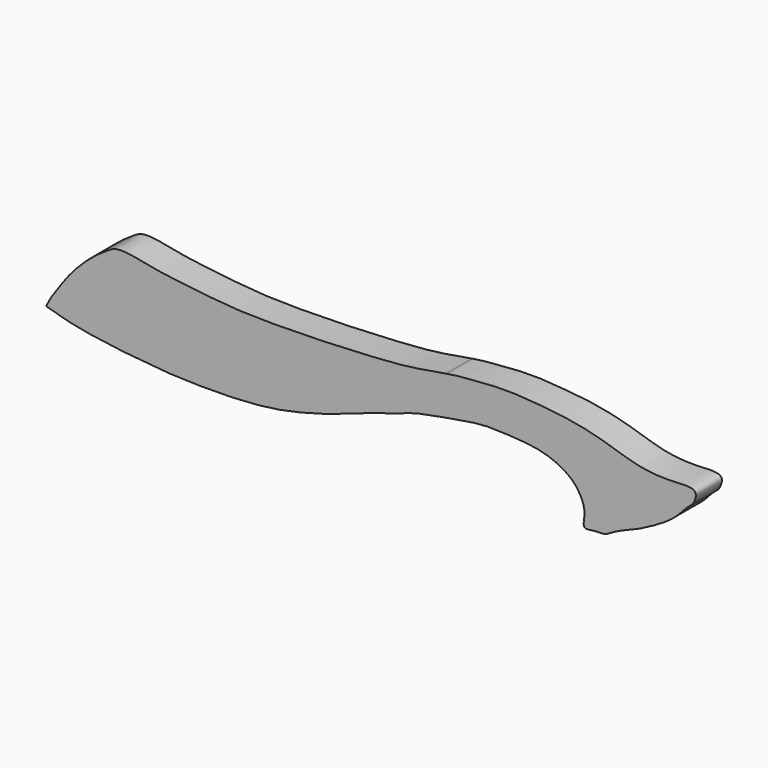
from build123d import *

# Parameters (mm, degrees)
F1_DEPTH = 25.4


with BuildPart() as f1:
    # F0 (on Front) → F1 (new body)
    with BuildSketch(Plane.XZ):
        with BuildLine():
            add(Edge.make_bspline(
                [(-41.3323794244, 51.0675903058), (-41.707539983, 51.0071643032), (-42.0874786851, 50.9453207608), (-42.4716510296, 50.8822327158)],
                knots=[0.7233820323, 0.7233820323, 0.7233820323, 0.7233820323, 0.7244841774, 0.7244841774, 0.7244841774, 0.7244841774], degree=3))
            Line((-42.4716510296, 50.8822327158), (-42.4716510296, 20.6025924894))
            add(Edge.make_bspline(
                [(-42.4716510296, 20.6025924894), (-38.0350865118, 21.387674424), (-27.1703671298, 23.2609805149), (-11.8336777596, 25.6290338302), (6.2117415006, 24.6446677805), (22.8981387265, 23.7685028967), (40.3803315985, 20.265824034), (56.0268632555, 11.4827913687), (63.3288722201, 1.5132508922), (67.2395318395, -9.5186102569), (63.4930685042, -21.7540557946), (73.9984795886, -18.6916156231), (82.1685298982, -19.9874563616), (89.9568581577, -13.8368079067), (103.8859155375, -9.029814598), (115.48254286, -3.1488551069), (127.3676268383, 3.4775298147), (138.3862701068, 11.274252363), (146.0514505158, 21.0054750541), (150.7100984849, 23.1711418755), (154.3469370428, 32.4931326622), (147.7952194183, 35.6662775706), (131.9063905367, 33.9551189768), (113.1540349234, 35.1939826272), (98.5720074401, 38.9368599863), (80.3169366587, 45.0640141502), (58.980025117, 50.1412876611), (38.6431779668, 52.6423918075), (18.2586858505, 54.3804757709), (-2.1281200842, 55.0935858146), (-25.7150036655, 52.83496744), (-33.7024906401, 52.247249559), (-39.6317656905, 51.3415031345), (-41.3323794244, 51.0675903058)],
                knots=[0.2661930696, 0.2661930696, 0.2661930696, 0.2661930696, 0.2780888488, 0.2952566157, 0.3124048676, 0.3290318413, 0.3462265461, 0.3632256959, 0.3773149803, 0.3913700519, 0.4035868461, 0.4147193685, 0.4265046687, 0.4388744688, 0.4544742419, 0.4692690904, 0.4841731354, 0.4993562758, 0.5132863243, 0.5226012229, 0.5341358793, 0.5434033522, 0.5596575999, 0.5774651553, 0.5931774764, 0.6109205173, 0.6300378187, 0.6484766733, 0.6666946566, 0.6854295214, 0.7048957488, 0.7183859765, 0.7233820323, 0.7233820323, 0.7233820323, 0.7233820323], degree=3))
        make_face()
        with BuildLine():
            Line((-42.4716510296, 20.6025924894), (-42.4716510296, 50.8822327158))
            add(Edge.make_bspline(
                [(-42.4716510296, 50.8822327158), (-46.5466181639, 50.2130494346), (-58.4983628647, 48.0880744628), (-77.3183947596, 45.1720060107), (-109.6591600511, 43.2576521666), (-142.7930612804, 41.7374006357), (-176.1120717601, 41.1768442804), (-208.717867936, 41.5632407424), (-242.6772032351, 45.6151659887), (-270.6437105384, 48.6410725006), (-297.2774912922, 55.186574868), (-306.7493706772, 49.342600006), (-316.6435316034, 42.6087777486), (-327.9751917318, 32.5628982927), (-337.3736197705, 21.5291356577), (-343.7111475225, 12.5988365582), (-348.0439396481, 6.508227293), (-349.970638752, 3.5016264301)],
                knots=[0.7244841774, 0.7244841774, 0.7244841774, 0.7244841774, 0.7361747771, 0.7551837741, 0.7782030276, 0.8018366623, 0.8252292117, 0.8485245896, 0.8721716095, 0.8943006879, 0.9149235119, 0.9278013284, 0.9416926123, 0.9576343562, 0.9731231453, 0.9865814519, 1, 1, 1, 1], degree=3))
            Line((-349.970638752, 3.5016264301), (-354.0885150433, -4.166085273))
            add(Edge.make_bspline(
                [(-354.0885150433, -4.166085273), (-350.9489476716, -5.1163888722), (-344.7462049827, -6.9958771891), (-329.8831910928, -10.712460005), (-315.9373628446, -12.9333647914), (-300.1678276103, -15.1690919729), (-289.0454983502, -16.3648427127), (-259.5457385506, -19.1871218728), (-240.3228415722, -19.9954402709), (-181.6003811838, -20.2349839719), (-140.814410437, -8.752844586), (-126.7065965954, -4.5985483975), (-103.1652458391, 4.5282060409), (-84.3034271709, 9.4039683704), (-68.3297105852, 15.8547238988), (-54.0010339859, 18.5393369104), (-44.9543762176, 20.1632564477), (-42.4716510296, 20.6025924894)],
                knots=[0, 0, 0, 0, 0.01268681, 0.0284135387, 0.0440599814, 0.0598488247, 0.0738522004, 0.0952719295, 0.1138868566, 0.1450282116, 0.171462617, 0.186967788, 0.2070464518, 0.2252615484, 0.2419043928, 0.259536128, 0.2661930696, 0.2661930696, 0.2661930696, 0.2661930696], degree=3))
        make_face()
    extrude(amount=F1_DEPTH)


solid = f1.part
